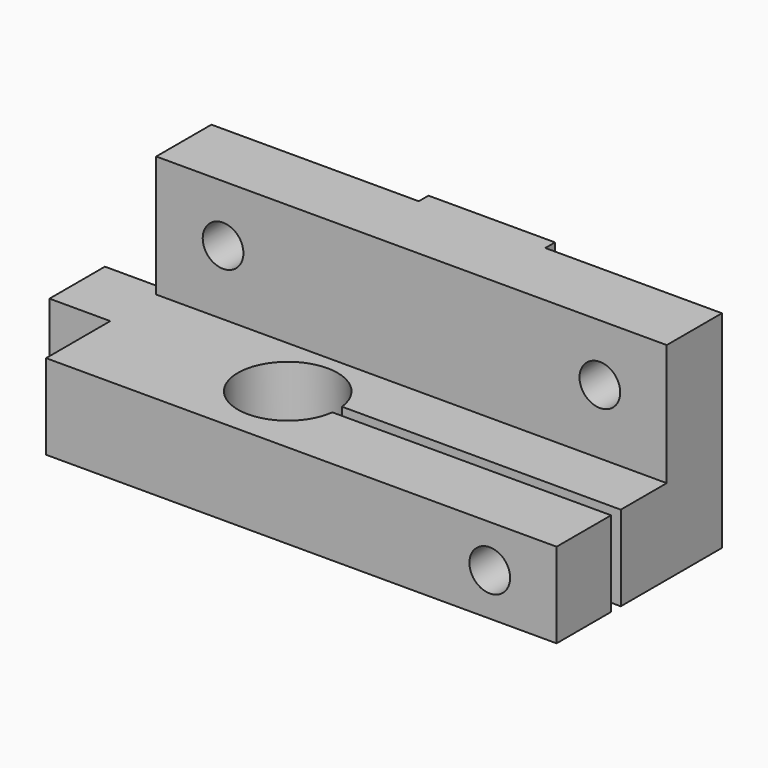
from build123d import *

# Parameters (mm, degrees)
F0_W          = 42
F0_H          = 17
F1_DEPTH      = 7
F4_DEPTH      = 25
F5_W          = 42
F5_H          = 5.6745335534
F6_DEPTH      = 10
F7_R          = 1.675
F8_DEPTH      = 25
F9_DEPTH      = 25
F10_TEXT_SIZE = 23.6111111111
F11_DEPTH     = 1
F12_W         = 5.7
F12_H         = 7
F13_DEPTH     = 5


# Not quite as in the source:
# - Text() gives the source's letters only with a copy of the font that has no kerning and outlines rounded to 1/6400 em; it was checked with that copy


with BuildPart() as f1:
    # F0 (on Top) → F1 (new body)
    with BuildSketch(Plane.XY):
        with Locations((21, 8.5)):
            Rectangle(F0_W, F0_H)
    extrude(amount=F1_DEPTH)

    # F3 (on face) → F4 (cut)
    with BuildSketch(Plane(origin=(0, 17, 0), x_dir=(-1, 0, 0), z_dir=(0, 1, 0))):
        with BuildLine():
            ThreePointArc((-38.175, 3.5), (-36.5, 1.825), (-34.825, 3.5))
            ThreePointArc((-34.825, 3.5), (-36.5, 5.175), (-38.175, 3.5))
        make_face()
    extrude(amount=-F4_DEPTH, mode=Mode.SUBTRACT)

    # F5 (on face) → F6 (join)
    with BuildSketch(Plane.XY.offset(7)):
        with Locations((21, 14.1627332233)):
            Rectangle(F5_W, F5_H)
    extrude(amount=F6_DEPTH)

    # F7 (on face) → F8 (cut)
    with BuildSketch(Plane(origin=(0, 17, 0), x_dir=(-1, 0, 0), z_dir=(0, 1, 0))):
        with Locations((-36.5, 12.325)):
            Circle(F7_R)
        with Locations((-5.5, 12.325)):
            Circle(F7_R)
    extrude(amount=-F8_DEPTH, mode=Mode.SUBTRACT)

    # F2 (on face) → F9 (cut)
    with BuildSketch(Plane.XY.offset(7)):
        with BuildLine():
            ThreePointArc((19.0693979899, 5.6), (19.0923423463, 5.8495321962), (19.1, 6.1))
            ThreePointArc((19.1, 6.1), (19.0923423463, 6.3504678038), (19.0693979899, 6.6))
            ThreePointArc((19.0693979899, 6.6), (10.9, 6.1), (19.0693979899, 5.6))
        make_face()
        with BuildLine():
            Line((42, 6.1), (19.1, 6.1))
            ThreePointArc((19.1, 6.1), (19.0923423463, 5.8495321962), (19.0693979899, 5.6))
            Line((19.0693979899, 5.6), (42, 5.6))
            Line((42, 5.6), (42, 6.1))
        make_face()
        with BuildLine():
            ThreePointArc((19.0693979899, 6.6), (19.0923423463, 6.3504678038), (19.1, 6.1))
            Line((19.1, 6.1), (42, 6.1))
            Line((42, 6.1), (42, 6.6))
            Line((42, 6.6), (19.0693979899, 6.6))
        make_face()
    extrude(amount=-F9_DEPTH, mode=Mode.SUBTRACT)

    # F10 (on face) → F11 (join)
    with BuildSketch(Plane(origin=(0, 17, 0), x_dir=(-1, 0, 0), z_dir=(0, 1, 0))):
        with Locations(Location((-14.9393391335, 17), (0, 0, -180))):
            Text('L', F10_TEXT_SIZE, font='Open Sans', font_style=FontStyle.BOLD, text_align=(TextAlign.LEFT, TextAlign.BOTTOM))
    extrude(amount=F11_DEPTH)

    # F12 (on face) → F13 (join)
    with BuildSketch(Plane(origin=(0, 0, 0), x_dir=(0, -1, 0), z_dir=(-1, 0, 0))):
        with Locations((-9.45, 3.5)):
            Rectangle(F12_W, F12_H)
    extrude(amount=F13_DEPTH)


solid = f1.part
